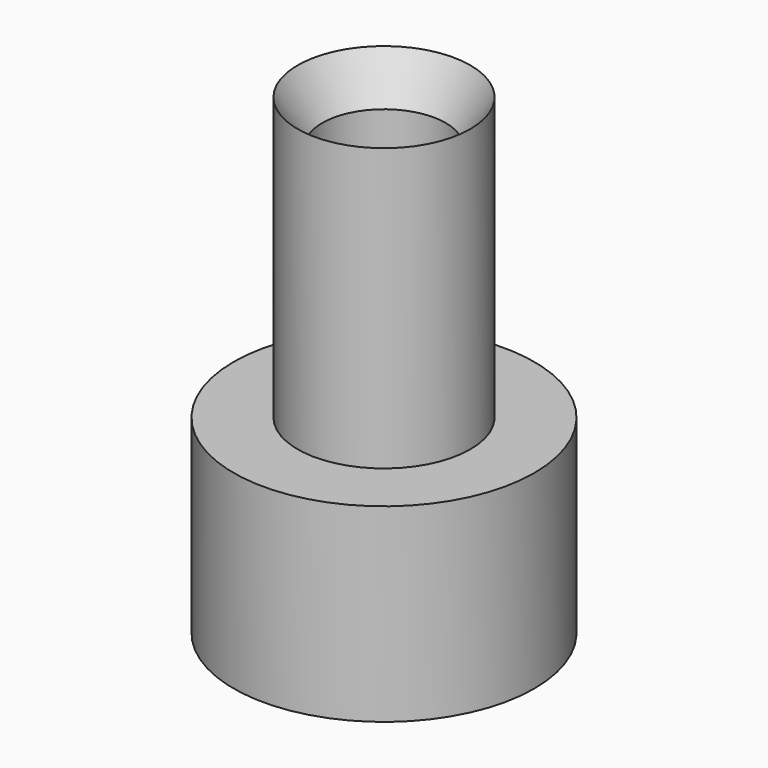
from build123d import *

# Parameters (mm, degrees)
F0_R     = 10.0595284502
F1_DEPTH = 12.7
F2_R     = 5.7785
F2_R_2   = 4.1275
F3_DEPTH = 19.05


# Not quite as in the source:
# - a fillet or chamfer that OpenCascade refuses, or shapes differently, is made with other operations: its cross-section is extruded or revolved along the edge and cut away or added


with BuildPart() as f1:
    # F0 (on Top) → F1 (new body)
    with BuildSketch(Plane.XY):
        Circle(F0_R)
    extrude(amount=F1_DEPTH)

    # F2 (on face) → F3 (join)
    with BuildSketch(Plane.XY.offset(12.7)):
        Circle(F2_R)
        Circle(F2_R_2, mode=Mode.SUBTRACT)
    extrude(amount=F3_DEPTH)

    # F4: chamfer of 3.048 x 1.7597636205 on 1 edges, made by hand

    # F4_s1 → F4_t2 (revolve, cut)
    with BuildSketch(Plane.XZ):
        Polygon((5.8872636205, 31.75), (4.1275, 28.702), (4.1275, 31.75), align=None)
    revolve(axis=Axis((0, 0, 31.75), (0, 0, 1)), mode=Mode.SUBTRACT)


solid = f1.part
